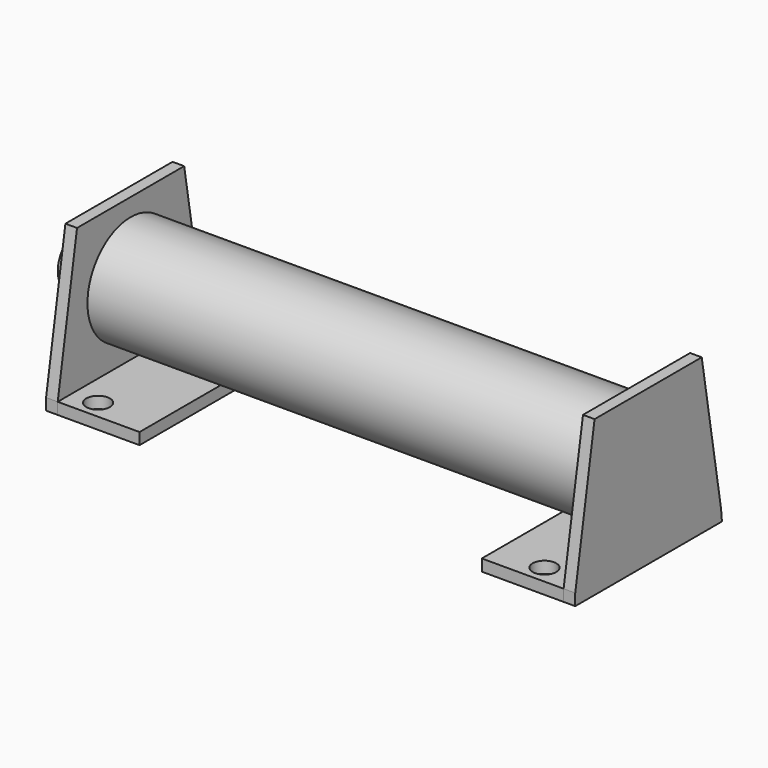
from build123d import *

# Parameters (mm, degrees)
F0_R      = 14.5034
F1_DEPTH  = 136
F2_R      = 6.9977
F3_DEPTH  = 13.9954
F5_DEPTH  = 22
F8_DEPTH  = 22
F9_DEPTH  = 3.1242
F11_DEPTH = 3.1242
F13_D     = 6.35
F13_2_D   = 6.35


# Not quite as in the source:
# - a feature names something its author has since deleted; it is built from what else it names


with BuildPart() as f1:
    # F0 (on Right) → F1 (new body)
    with BuildSketch(Plane.YZ):
        Circle(F0_R)
    extrude(amount=F1_DEPTH)


with BuildPart() as f3:
    # F2 (on Right) → F3 (new body)
    with BuildSketch(Plane.YZ):
        Circle(F2_R)
    extrude(amount=-F3_DEPTH)


with BuildPart() as f5:
    # F4 (on Right) → F5 (new body)
    with BuildSketch(Plane.YZ):
        Polygon((24.5, -19.25), (0, -19.25), (-24.5, -19.25), (-24.5, -22.3650014941), (24.5, -22.3650014941), align=None)
    extrude(amount=F5_DEPTH)

    # F13 (through all)
    with Locations(Plane.XY.offset(-19.25)):
        with Locations((6.8870979548, -19.5322781801), (6.8870979548, 20.4677218199), (126.8870979548, 20.4677218199), (126.8870979548, -19.5322781801)):
            Hole(F13_D / 2)


with BuildPart() as f8:
    # F7 (on offset) → F8 (new body)
    with BuildSketch(Plane.YZ.offset(136)):
        Polygon((0, -19.25), (-24.5, -19.25), (-24.5, -22.3742), (24.7841487321, -22.3742), (24.5, -19.25), align=None)
    extrude(amount=-F8_DEPTH)

    # F13#2 (through all)
    with Locations(Plane.XY.offset(-19.25)):
        with Locations((6.8870979548, -19.5322781801), (6.8870979548, 20.4677218199), (126.8870979548, 20.4677218199), (126.8870979548, -19.5322781801)):
            Hole(F13_2_D / 2)


with BuildPart() as f9:
    # F7 (on offset) → F9 (new body)
    with BuildSketch(Plane.YZ.offset(136)):
        Polygon((0, 19.25), (-18, 19.25), (-24.5, -19.25), (0, -19.25), align=None)
        Polygon((18, 19.25), (0, 19.25), (0, -19.25), (24.5, -19.25), align=None)
        Polygon((0, -19.25), (-24.5, -19.25), (-24.5, -22.3742), (24.7841487321, -22.3742), (24.5, -19.25), align=None)
    extrude(amount=F9_DEPTH)


with BuildPart() as f11:
    # F4 (on Right) → F11 (new body)
    with BuildSketch(Plane.YZ):
        Polygon((18, 19.25), (0, 19.25), (0, -19.25), (24.5, -19.25), align=None)
        Polygon((0, -19.25), (0, 19.25), (-18, 19.25), (-24.5, -19.25), align=None)
        Polygon((24.5, -19.25), (0, -19.25), (-24.5, -19.25), (-24.5, -22.3650014941), (24.5, -22.3650014941), align=None)
    extrude(amount=-F11_DEPTH)


solid = Compound([f1.part, f3.part, f5.part, f8.part, f9.part, f11.part])
